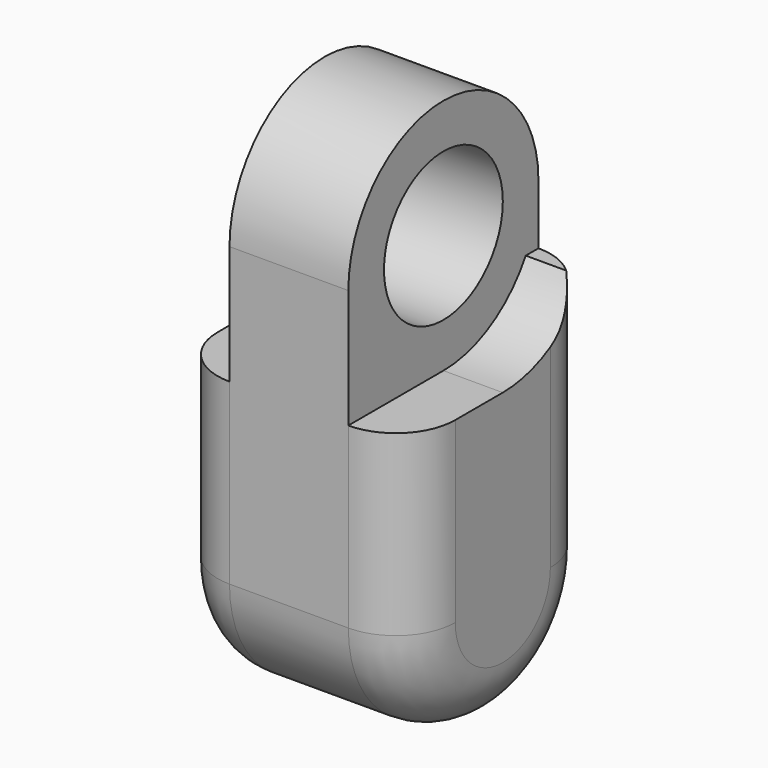
from build123d import *

# Parameters (mm, degrees)
F0_R     = 1.25
F1_DEPTH = 2
F3_DEPTH = 1
F5_R     = 1


# Not quite as in the source:
# - a pattern or mirror of a feature is missing from the dataset's text; its kind, count and spacing are read off the source's solid


with BuildPart() as f1:
    # F0 (on Right) → F1 (new body)
    with BuildSketch(Plane.YZ):
        with BuildLine():
            ThreePointArc((-2, 0), (0, -2), (2, 0))
            ThreePointArc((2, 0), (0, 2), (-2, 0))
        make_face()
        Circle(F0_R, mode=Mode.SUBTRACT)
        with BuildLine():
            Line((2, -5), (2, 0))
            ThreePointArc((2, 0), (0, -2), (-2, 0))
            Line((-2, 0), (-2, -5))
            ThreePointArc((-2, -5), (0, -3), (2, -5))
        make_face()
        with BuildLine():
            ThreePointArc((-2, -5), (0, -7), (2, -5))
            Line((2, -5), (-2, -5))
        make_face()
        with BuildLine():
            Line((-2, -5), (2, -5))
            ThreePointArc((2, -5), (0, -3), (-2, -5))
        make_face()
    extrude(amount=-F1_DEPTH)

    # F2 (on face) → F3 (join)
    with BuildSketch(Plane(origin=(-2, 0, 0), x_dir=(0, -1, 0), z_dir=(-1, 0, 0))):
        with BuildLine():
            ThreePointArc((0, -2), (-1, -1.7320508076), (-1.7320508076, -1))
            Line((-1.7320508076, -1), (-2, -1))
            Line((-2, -1), (-2, -4))
            Line((-2, -4), (-1.7320508076, -4))
            ThreePointArc((-1.7320508076, -4), (-1, -3.2679491924), (0, -3))
            Line((0, -3), (2, -3))
            Line((2, -3), (2, -2))
            Line((2, -2), (0, -2))
        make_face()
        with BuildLine():
            Line((-1.7320508076, -4), (-2, -4))
            Line((-2, -4), (-2, -5))
            ThreePointArc((-2, -5), (0, -7), (2, -5))
            Line((2, -5), (2, -3))
            Line((2, -3), (0, -3))
            ThreePointArc((0, -3), (-1, -3.2679491924), (-1.7320508076, -4))
        make_face()
    f3 = extrude(amount=F3_DEPTH)

    # F3_copies: F3 across plane
    add(f3.mirror(Plane(origin=(-1, 0, 0), x_dir=(0, 0, 1), z_dir=(1, 0, 0))))

    # F5
    f5_edges = [f1.edges().sort_by_distance(p)[0] for p in [
        (-3, 2, -3),
        (-3, -2, -3.5),
        (-3, 0, -7),
        (1, 0, -7),
        (1, 2, -3),
        (1, -2, -3.5),
    ]]
    fillet(f5_edges, radius=F5_R)


solid = f1.part
